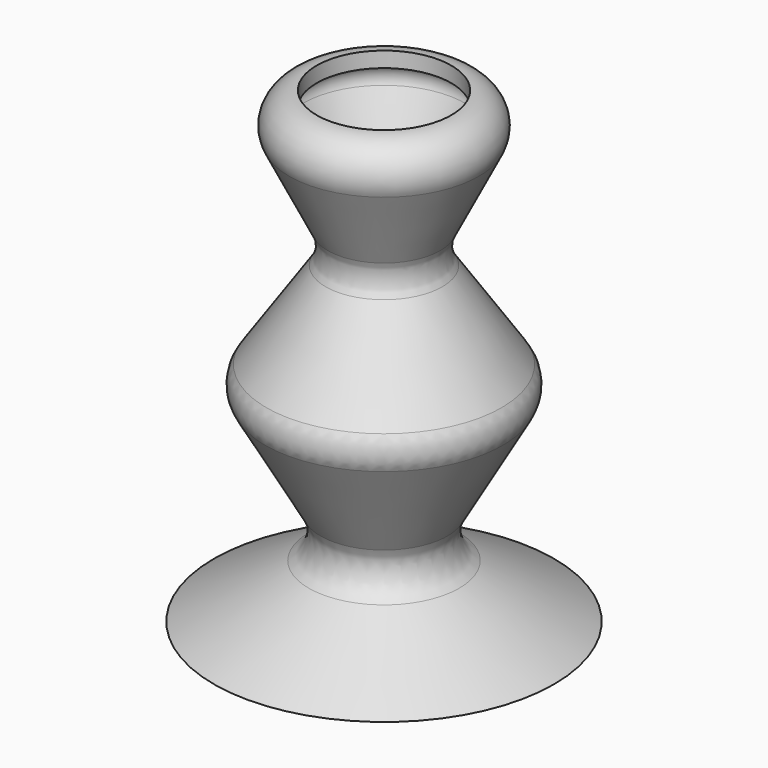
from build123d import *

# Parameters (mm, degrees)
F2_R = 5.08
F3_T = -2.54


# Not quite as in the source:
# - a shell that OpenCascade refuses in one call is made with other operations: the cavity is built on its own and cut out


with BuildPart() as f1:
    # F0 (on Front) → F1 (revolve)
    with BuildSketch(Plane.XZ):
        Polygon((-27.9191825539, -76.7777636647), (0, -76.7777636647), (0, 0), (-19.2415993661, 0), (-7.923011668, -22.8258222342), (-21.0848007405, -42.2066817869), (-7.923011668, -65.459176898), align=None)
    revolve(axis=Axis((0, 0, -38.3888818324), (0, 0, -1)))

    # F2
    f2_edges = [f1.edges().sort_by_distance(p)[0] for p in [
        (21.084801, 0, -42.206682),
        (7.923012, 0, -22.825822),
        (19.241599, 0, 0),
        (-13.582306, 0, -11.412911),
        (7.923012, 0, -65.459177),
    ]]
    fillet(f2_edges, radius=F2_R)

    # F3: a shell. OpenCascade refuses it in one call, so the cavity is built on its own and cut out:
    # the body offset inwards by the wall thickness, plus a prism from it out through each open face.
    f3_core = offset(f1.part, amount=F3_T, mode=Mode.PRIVATE)
    f3_exits = [f3_core.faces().sort_by_distance(p)[0] for p in [
        (0, 0, -2.54),
    ]]
    add(f3_core, mode=Mode.SUBTRACT)
    extrude(f3_exits, amount=-F3_T, mode=Mode.SUBTRACT)


solid = f1.part
